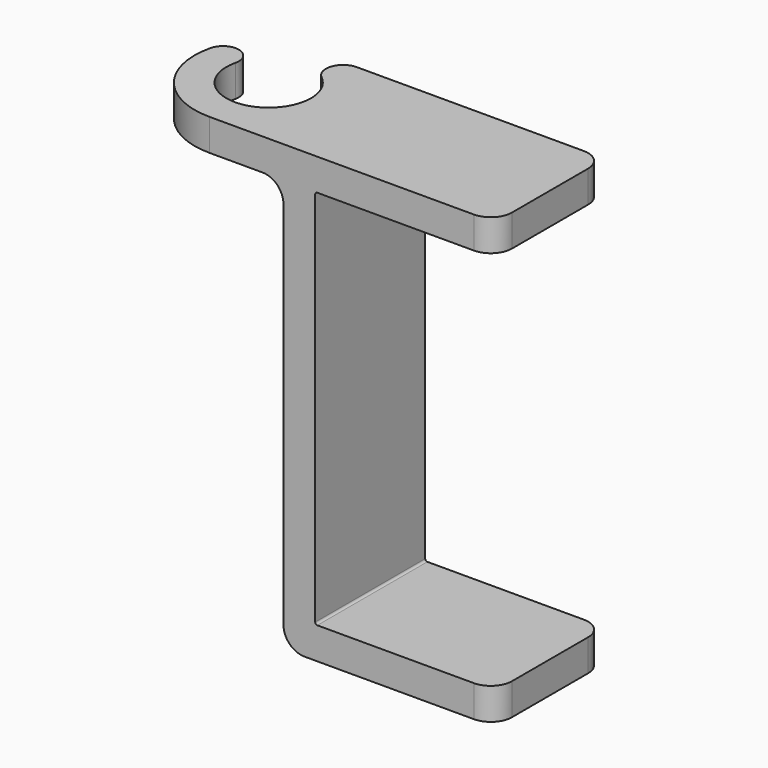
from build123d import *

# Parameters (mm, degrees)
F1_DEPTH = 1.5
F3_DEPTH = 6.5
F4_R     = 0.1
F5_R     = 1
F6_R     = 1


# Not quite as in the source:
# - a feature of the source that left no trace in its solid (it failed there, or was rolled back) is left out


with BuildPart() as f1:
    # F0 (on Top) → F1 (new body)
    with BuildSketch(Plane.XY):
        with BuildLine():
            Line((13.5, -3.5), (13.5, 3))
            Line((13.5, 3), (1.7699947357, 3))
            ThreePointArc((1.7699947357, 3), (1.00332674, 2.4581115268), (1.2583103115, 1.5545594745))
            ThreePointArc((1.2583103115, 1.5545594745), (0.6431264076, -1.8937762339), (-1.9447626006, 0.466795916))
            ThreePointArc((-1.9447626006, 0.466795916), (-2.4990001073, 1.3711303598), (-3.4033345511, 0.8168928531))
            ThreePointArc((-3.4033345511, 0.8168928531), (-2.748556438, -2.1668958229), (0, -3.5))
            Line((0, -3.5), (1.7699947357, -3.5))
            Line((1.7699947357, -3.5), (13.5, -3.5))
        make_face()
    extrude(amount=F1_DEPTH)

    # F2 (on face) → F3 (join, through all)
    with BuildSketch(Plane.XZ.offset(3.5)):
        Polygon((5, 0), (3.5, 0), (3.5, -19.5), (13.5, -19.5), (13.5, -18), (5, -18), align=None)
    extrude(amount=-F3_DEPTH)

    # F4
    f4_edges = [f1.edges().sort_by_distance(p)[0] for p in [
        (5, -0.25, 0),
        (5, -0.25, -18),
    ]]
    fillet(f4_edges, radius=F4_R)

    # F5
    f5_edges = [f1.edges().sort_by_distance(p)[0] for p in [
        (3.5, -0.25, 0),
        (3.5, -0.25, -19.5),
    ]]
    fillet(f5_edges, radius=F5_R)

    # F6
    f6_edges = [f1.edges().sort_by_distance(p)[0] for p in [
        (13.5, -3.5, -18.75),
        (13.5, 3, -18.75),
        (13.5, -3.5, 0.75),
        (13.5, 3, 0.75),
    ]]
    fillet(f6_edges, radius=F6_R)


solid = f1.part
